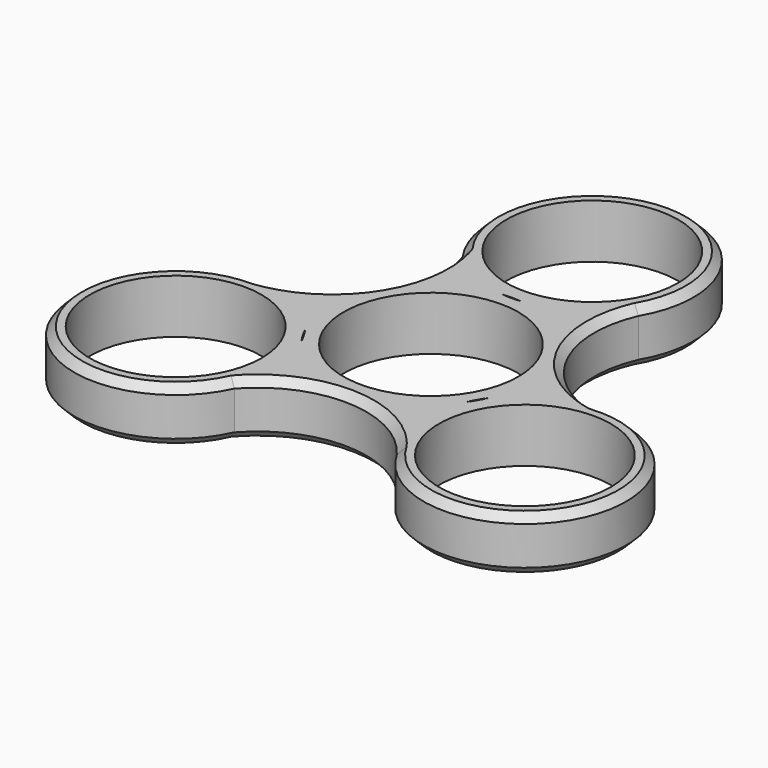
from build123d import *

# Parameters (mm, degrees)
F0_R        = 11.15
F0_R_2      = 11.35
F1_DEPTH    = 7
F2_C1_SIZE  = 1
F2_C2_SIZE  = 1
F2_C3_SIZE  = 1
F2_C4_SIZE  = 1
F2_C5_SIZE  = 1
F2_C6_SIZE  = 1
F2_C7_SIZE  = 0.9999
F2_C8_SIZE  = 0.9999
F2_C9_SIZE  = 0.9999
F2_C10_SIZE = 0.9999
F2_C11_SIZE = 0.9999
F2_C12_SIZE = 0.9999


# Not quite as in the source:
# - a fillet or chamfer is up to 0.001 mm smaller than in the source, because OpenCascade refuses the exact size


with BuildPart() as f1:
    # F0 (on Top) → F1 (new body)
    with BuildSketch(Plane.XY):
        with BuildLine():
            ThreePointArc((21.4042818528, 0), (11.7146810466, 7.3545646083), (11.3361036393, 19.5132924821))
            ThreePointArc((11.3361036393, 19.5132924821), (-0.5821803149, 39.3148759845), (-10.7021409264, 18.5366518343))
            ThreePointArc((-10.7021409264, 18.5366518343), (-12.2265803079, 6.4679290794), (-22.5670588206, 0.0607074905))
            ThreePointArc((-22.5670588206, 0.0607074905), (-33.7565911918, -20.1616209346), (-10.7021409264, -18.5366518343))
            ThreePointArc((-10.7021409264, -18.5366518343), (0.5118992613, -13.8224936877), (11.2309551813, -19.5739999726))
            ThreePointArc((11.2309551813, -19.5739999726), (34.3387715067, -19.15325505), (21.4042818528, 0))
        make_face()
        with Locations((-22.6706134247, -13.0888847634)):
            Circle(F0_R, mode=Mode.SUBTRACT)
        with BuildLine():
            ThreePointArc((-11.9684724983, -5.4477670709), (-11.2823793649, -6.5138847634), (-10.7021409264, -7.6411176926))
            ThreePointArc((-10.7021409264, -7.6411176926), (-11.3882340598, -6.575), (-11.9684724983, -5.4477670709))
        make_face(mode=Mode.SUBTRACT)
        with Locations((22.6706134247, -13.0888847634)):
            Circle(F0_R, mode=Mode.SUBTRACT)
        with BuildLine():
            ThreePointArc((11.9684724983, -5.4477670709), (11.3882340598, -6.575), (10.7021409264, -7.6411176926))
            ThreePointArc((10.7021409264, -7.6411176926), (11.2823793649, -6.5138847634), (11.9684724983, -5.4477670709))
        make_face(mode=Mode.SUBTRACT)
        Circle(F0_R_2, mode=Mode.SUBTRACT)
        with BuildLine():
            ThreePointArc((-1.2663315719, 13.0888847634), (0, 13.15), (1.2663315719, 13.0888847634))
            ThreePointArc((1.2663315719, 13.0888847634), (0, 13.0277695268), (-1.2663315719, 13.0888847634))
        make_face(mode=Mode.SUBTRACT)
        with Locations((0, 26.1777695268)):
            Circle(F0_R, mode=Mode.SUBTRACT)
    extrude(amount=F1_DEPTH)

    # F2: chamfer of 1 on 12 edges, made by hand

    # F2_c1
    f2_c1_edges = [f1.edges().sort_by_distance(p)[0] for p in [
        (0.5118992613, -13.8224936877, 0),
    ]]
    chamfer(f2_c1_edges, length=F2_C1_SIZE)

    # F2_c2
    f2_c2_edges = [f1.edges().sort_by_distance(p)[0] for p in [
        (0.5118992613, -13.8224936877, 7),
    ]]
    chamfer(f2_c2_edges, length=F2_C2_SIZE)

    # F2_c3
    f2_c3_edges = [f1.edges().sort_by_distance(p)[0] for p in [
        (11.7146810466, 7.3545646083, 0),
    ]]
    chamfer(f2_c3_edges, length=F2_C3_SIZE)

    # F2_c4
    f2_c4_edges = [f1.edges().sort_by_distance(p)[0] for p in [
        (11.7146810466, 7.3545646083, 7),
    ]]
    chamfer(f2_c4_edges, length=F2_C4_SIZE)

    # F2_c5
    f2_c5_edges = [f1.edges().sort_by_distance(p)[0] for p in [
        (-12.2265803079, 6.4679290794, 0),
    ]]
    chamfer(f2_c5_edges, length=F2_C5_SIZE)

    # F2_c6
    f2_c6_edges = [f1.edges().sort_by_distance(p)[0] for p in [
        (-12.2265803079, 6.4679290794, 7),
    ]]
    chamfer(f2_c6_edges, length=F2_C6_SIZE)

    # F2_c7 (size 1 in the source; OpenCascade refuses exactly that, so slightly less here)
    f2_c7_edges = [f1.edges().sort_by_distance(p)[0] for p in [
        (-33.7565911918, -20.1616209346, 0),
    ]]
    chamfer(f2_c7_edges, length=F2_C7_SIZE)

    # F2_c8 (size 1 in the source; OpenCascade refuses exactly that, so slightly less here)
    f2_c8_edges = [f1.edges().sort_by_distance(p)[0] for p in [
        (-33.7565911918, -20.1616209346, 7),
    ]]
    chamfer(f2_c8_edges, length=F2_C8_SIZE)

    # F2_c9 (size 1 in the source; OpenCascade refuses exactly that, so slightly less here)
    f2_c9_edges = [f1.edges().sort_by_distance(p)[0] for p in [
        (34.3387715067, -19.15325505, 0),
    ]]
    chamfer(f2_c9_edges, length=F2_C9_SIZE)

    # F2_c10 (size 1 in the source; OpenCascade refuses exactly that, so slightly less here)
    f2_c10_edges = [f1.edges().sort_by_distance(p)[0] for p in [
        (34.3387715067, -19.15325505, 7),
    ]]
    chamfer(f2_c10_edges, length=F2_C10_SIZE)

    # F2_c11 (size 1 in the source; OpenCascade refuses exactly that, so slightly less here)
    f2_c11_edges = [f1.edges().sort_by_distance(p)[0] for p in [
        (-0.5821803149, 39.3148759845, 0),
    ]]
    chamfer(f2_c11_edges, length=F2_C11_SIZE)

    # F2_c12 (size 1 in the source; OpenCascade refuses exactly that, so slightly less here)
    f2_c12_edges = [f1.edges().sort_by_distance(p)[0] for p in [
        (-0.5821803149, 39.3148759845, 7),
    ]]
    chamfer(f2_c12_edges, length=F2_C12_SIZE)


solid = f1.part
